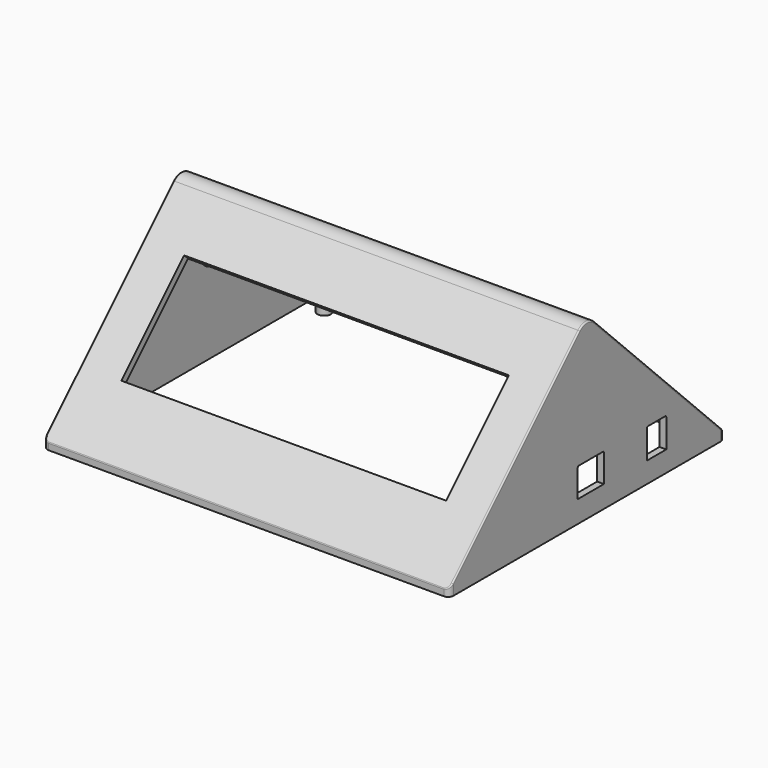
from build123d import *

# Parameters (mm, degrees)
F1_DEPTH  = 150
F2_T      = -2.5
F4_W      = 120
F4_H      = 41
F5_DEPTH  = 3
F6_R      = 5
F8_R      = 1.5
F8_R_2    = 0.75
F9_DEPTH  = 6.5
F10_R     = 2.5
F10_R_2   = 1.5
F12_R     = 2.5
F12_R_2   = 1.25
F13_REACH = 68.6406103068
F14_W     = 150
F14_H     = 127.2792206136
F14_W_2   = 145
F14_H_2   = 120.2081528017
F15_DEPTH = 2.5
F16_R     = 2.5
F16_R_2   = 1.25
F18_R     = 2
F19_R     = 0.5
F7_W      = 9
F7_H      = 11
F7_W_2    = 12.1
F7_H_2    = 10.7
F20_DEPTH = 3
F21_R     = 0.5
F22_R     = 0.5
F23_R     = 6.5
F24_DEPTH = 2.5
F25_R     = 2.5
F25_R_2   = 1.25
F26_DEPTH = 2.5


with BuildPart() as f1:
    # F0 (on Right) → F1 (new body)
    with BuildSketch(Plane.YZ):
        Polygon((63.6396103068, 63.6396103068), (0, 0), (127.2792206136, 0), align=None)
    extrude(amount=F1_DEPTH)

    # F2
    f2_openings = [f1.faces().sort_by_distance(p)[0] for p in [
        (75, 63.63961, 0),
    ]]
    offset(amount=F2_T, openings=f2_openings, kind=Kind.INTERSECTION)

    # F4 (on offset) → F5 (cut)
    with BuildSketch(Plane(origin=(0, 0, 0), x_dir=(1, 0, 0), z_dir=(0, -0.7071067812, 0.7071067812))):
        with Locations((75, 45)):
            Rectangle(F4_W, F4_H)
    extrude(amount=-F5_DEPTH, mode=Mode.SUBTRACT)

    # F6
    f6_edges = [f1.edges().sort_by_distance(p)[0] for p in [
        (75, 63.63961, 63.63961),
    ]]
    fillet(f6_edges, radius=F6_R)

    # F8 (on face) → F9 (join)
    with BuildSketch(Plane(origin=(0, 0, 0), x_dir=(1, 0, 0), z_dir=(0, -0.7071067812, 0.7071067812))):
        with Locations((131, 67.5)):
            Circle(F8_R)
        with Locations((131, 67.5)):
            Circle(F8_R_2, mode=Mode.SUBTRACT)
        with Locations((131, 22.5)):
            Circle(F8_R)
        with Locations((131, 22.5)):
            Circle(F8_R_2, mode=Mode.SUBTRACT)
        with Locations((19, 67.5)):
            Circle(F8_R)
        with Locations((19, 67.5)):
            Circle(F8_R_2, mode=Mode.SUBTRACT)
        with Locations((19, 22.5)):
            Circle(F8_R)
        with Locations((19, 22.5)):
            Circle(F8_R_2, mode=Mode.SUBTRACT)
    extrude(amount=-F9_DEPTH)

    # F10 (on face) → F11 (join, up to the last surface of F1)
    with BuildSketch(Plane(origin=(0, 0, 0), x_dir=(1, 0, 0), z_dir=(0, 0, -1))):
        with Locations((10, -10)):
            Circle(F10_R)
        with Locations((10, -10)):
            Circle(F10_R_2, mode=Mode.SUBTRACT)
    extrude(until=Until.LAST, dir=(0, 0, 1))

    f13_end = Plane(origin=(75.2456023398, 33.6766976894, 30.1411637835), x_dir=(0, 0.7071067812, 0.7071067812), z_dir=(0, 0.7071067812, -0.7071067812))
    # F12 (on face) → F13 (join, up to a plane its end follows)
    with BuildSketch(Plane(origin=(0, 0, 0), x_dir=(1, 0, 0), z_dir=(0, 0, -1))):
        with Locations((10, -10)):
            Circle(F12_R)
        with Locations((10, -10)):
            Circle(F12_R_2, mode=Mode.SUBTRACT)
        with Locations((140, -10)):
            Circle(F12_R)
        with Locations((140, -10)):
            Circle(F12_R_2, mode=Mode.SUBTRACT)
    f13_long = extrude(amount=-F13_REACH, mode=Mode.PRIVATE)
    add(split(f13_long, bisect_by=f13_end, keep=Keep.TOP, mode=Mode.PRIVATE))

    # F14 (on face) → F15 (join)
    with BuildSketch(Plane(origin=(0, 0, 0), x_dir=(1, 0, 0), z_dir=(0, 0, -1))):
        with Locations((75, -63.6396103068)):
            Rectangle(F14_W, F14_H)
        with Locations((75, -63.6396103068)):
            Rectangle(F14_W_2, F14_H_2, mode=Mode.SUBTRACT)
    extrude(amount=F15_DEPTH)

    # F16 (on Top) → F17 (join, up to the next surface of F1)
    with BuildSketch(Plane.XY):
        with Locations((140, 117.279)):
            Circle(F16_R)
        with Locations((140, 117.279)):
            Circle(F16_R_2, mode=Mode.SUBTRACT)
        with Locations((10, 117.279)):
            Circle(F16_R)
        with Locations((10, 117.279)):
            Circle(F16_R_2, mode=Mode.SUBTRACT)
    extrude(until=Until.NEXT)

    # F18
    f18_edges = [f1.edges().sort_by_distance(p)[0] for p in [
        (150, 127.279221, -1.25),
        (150, 0, -1.25),
        (0, 0, -1.25),
        (0, 127.279221, -1.25),
    ]]
    fillet(f18_edges, radius=F18_R)

    # F19
    f19_edges = [f1.edges().sort_by_distance(p)[0] for p in [
        (0, 31.052038, 31.052038),
    ]]
    fillet(f19_edges, radius=F19_R)

    # F7 (on face) → F20 (cut)
    with BuildSketch(Plane.YZ.offset(150)):
        with Locations((95.7792206136, 10.65)):
            Rectangle(F7_W, F7_H)
        with Locations((65.4042206136, 10.95)):
            Rectangle(F7_W_2, F7_H_2)
    extrude(amount=-F20_DEPTH, mode=Mode.SUBTRACT)

    # F21
    f21_edges = [f1.edges().sort_by_distance(p)[0] for p in [
        (148.75, 91.279221, 16.15),
        (148.75, 100.279221, 16.15),
    ]]
    fillet(f21_edges, radius=F21_R)

    # F22
    f22_edges = [f1.edges().sort_by_distance(p)[0] for p in [
        (148.75, 59.354221, 16.3),
        (148.75, 71.454221, 16.3),
    ]]
    fillet(f22_edges, radius=F22_R)

    # F23 (on face) → F24 (cut)
    with BuildSketch(Plane(origin=(0, 0, 0), x_dir=(0, -1, 0), z_dir=(-1, 0, 0))):
        with Locations((-64, 47.5)):
            Circle(F23_R)
    extrude(amount=-F24_DEPTH, mode=Mode.SUBTRACT)

    # F25 (on face) → F26 (join)
    with BuildSketch(Plane(origin=(0, 0, 0), x_dir=(1, 0, 0), z_dir=(0, 0, -1))):
        with Locations((10, -10)):
            Circle(F25_R)
        with Locations((10, -10)):
            Circle(F25_R_2, mode=Mode.SUBTRACT)
        with Locations((140, -10)):
            Circle(F25_R)
        with Locations((140, -10)):
            Circle(F25_R_2, mode=Mode.SUBTRACT)
        with Locations((10, -117.279)):
            Circle(F25_R)
        with Locations((10, -117.279)):
            Circle(F25_R_2, mode=Mode.SUBTRACT)
        with Locations((140, -117.279)):
            Circle(F25_R)
        with Locations((140, -117.279)):
            Circle(F25_R_2, mode=Mode.SUBTRACT)
    extrude(amount=F26_DEPTH)


solid = f1.part
